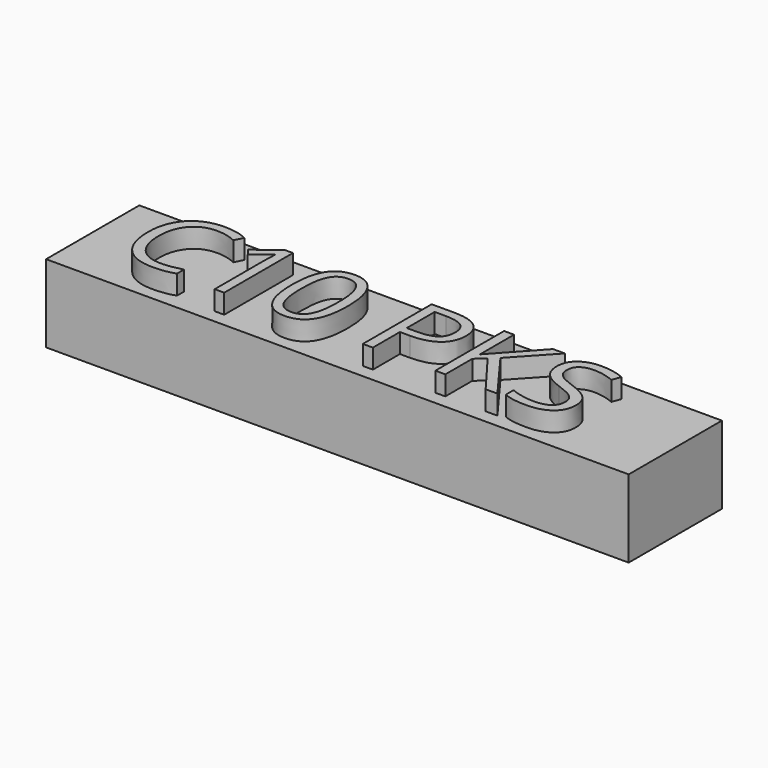
from build123d import *

# Parameters (mm, degrees)
F0_W         = 30
F0_H         = 6
F1_DEPTH     = 4
F2_TEXT_SIZE = 6.1967410147
F3_DEPTH     = 1
F4_DEPTH     = 4


# Not quite as in the source:
# - a feature of the source that left no trace in its solid (it failed there, or was rolled back) is left out
# - Text() gives the source's letters only with a copy of the font that has no kerning and outlines rounded to 1/6400 em; it was checked with that copy


with BuildPart() as f1:
    # F0 (on Top) → F1 (new body)
    with BuildSketch(Plane.XY):
        with Locations((-29.1523613761, 47.5559318438)):
            Rectangle(F0_W, F0_H)
    extrude(amount=F1_DEPTH)


with BuildPart() as f3:
    # F2 (on face) → F3 (new body)
    with BuildSketch(Plane.XY.offset(4)):
        with Locations((-41.6100472212, 45.2519133687)):
            Text('C10 PKS', F2_TEXT_SIZE, font='Open Sans', text_align=(TextAlign.LEFT, TextAlign.BOTTOM))
    extrude(amount=F3_DEPTH)


with BuildPart() as f4:
    # F0 (on Top) → F4 (new body)
    with BuildSketch(Plane.XY):
        with Locations((-29.1523613761, 47.5559318438)):
            Rectangle(F0_W, F0_H)
    extrude(amount=F4_DEPTH)


solid = Compound([f1.part, f3.part, f4.part])
